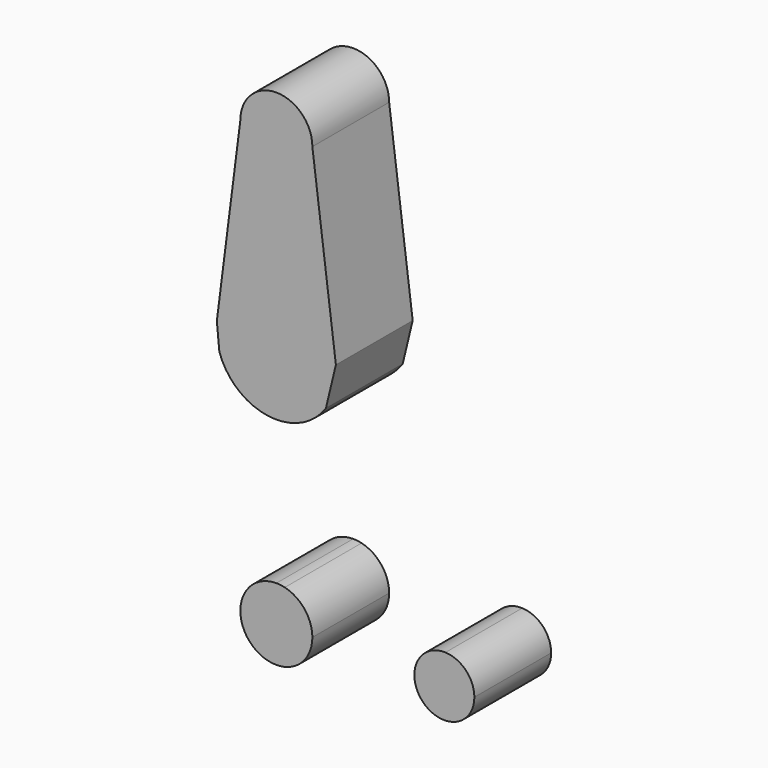
from build123d import *

# Parameters (mm, degrees)
F1_DEPTH = 25.4


# Not quite as in the source:
# - a feature names something its author has since deleted; it is built from what else it names


with BuildPart() as f1:
    # F0 (on Front) → F1 (new body)
    with BuildSketch(Plane.XZ):
        with BuildLine():
            ThreePointArc((0, 104.775), (6.7351920908, 107.5648079092), (9.525, 114.3))
            ThreePointArc((9.525, 114.3), (0, 123.825), (-9.525, 114.3))
            ThreePointArc((-9.525, 114.3), (-6.7351920908, 107.5648079092), (0, 104.775))
        make_face()
        with BuildLine():
            Line((15.7474569047, 65.5082893304), (9.525, 114.3))
            ThreePointArc((9.525, 114.3), (6.7351920908, 107.5648079092), (0, 104.775))
            Line((0, 104.775), (0, 79.375))
            ThreePointArc((0, 79.375), (10.4912828548, 75.4142187767), (15.7474569047, 65.5082893304))
        make_face()
        with BuildLine():
            ThreePointArc((0, 104.775), (-6.7351920908, 107.5648079092), (-9.525, 114.3))
            Line((-9.525, 114.3), (-15.7474569047, 65.5082893304))
            ThreePointArc((-15.7474569047, 65.5082893304), (-10.4912828548, 75.4142187767), (0, 79.375))
            Line((0, 79.375), (0, 104.775))
        make_face()
        with BuildLine():
            Line((13.1141006333, 54.5537164375), (15.7474569047, 65.5082893304))
            ThreePointArc((15.7474569047, 65.5082893304), (10.4912828548, 75.4142187767), (0, 79.375))
            ThreePointArc((0, 79.375), (-10.4912828548, 75.4142187767), (-15.7474569047, 65.5082893304))
            Line((-15.7474569047, 65.5082893304), (-15.0940259351, 58.5820729906))
            ThreePointArc((-15.0940259351, 58.5820729906), (-2.2443128525, 47.7844444953), (13.1141006333, 54.5537164375))
        make_face()
    extrude(amount=F1_DEPTH)


with BuildPart() as f1b:
    # F0 (on Front) → F1, piece 2 (new body)
    with BuildSketch(Plane.XZ):
        with BuildLine():
            Line((0, -9.525), (0.6773435479, -9.500885786))
            ThreePointArc((0.6773435479, -9.500885786), (6.9705567315, -6.4912990883), (9.525, 0))
            Line((9.525, 0), (0, 0))
            Line((0, 0), (0, 9.525))
            ThreePointArc((0, 9.525), (-9.525, 0), (0, -9.525))
        make_face()
        with BuildLine():
            Line((0, 0), (9.525, 0))
            ThreePointArc((9.525, 0), (7.4810078517, 5.8957736152), (2.2262815701, 9.2611713822))
            Line((2.2262815701, 9.2611713822), (0, 0))
        make_face()
        with BuildLine():
            ThreePointArc((2.2262815701, 9.2611713822), (1.1209298784, 9.4588128858), (0, 9.525))
            Line((0, 9.525), (0, 0))
            Line((0, 0), (2.2262815701, 9.2611713822))
        make_face()
    extrude(amount=F1_DEPTH)


with BuildPart() as f1c:
    # F0 (on Front) → F1, piece 3 (new body)
    with BuildSketch(Plane.XZ):
        with BuildLine():
            ThreePointArc((52.3875, 0), (50.1616327839, 5.5119104847), (44.7324052746, 7.9324746146))
            ThreePointArc((44.7324052746, 7.9324746146), (38.9380895153, 5.7116327839), (36.5125, 0))
            ThreePointArc((36.5125, 0), (38.9380895153, -5.7116327839), (44.7324052746, -7.9324746146))
            ThreePointArc((44.7324052746, -7.9324746146), (50.1616327839, -5.5119104847), (52.3875, 0))
        make_face()
    extrude(amount=F1_DEPTH)


solid = Compound([f1.part, f1b.part, f1c.part])
